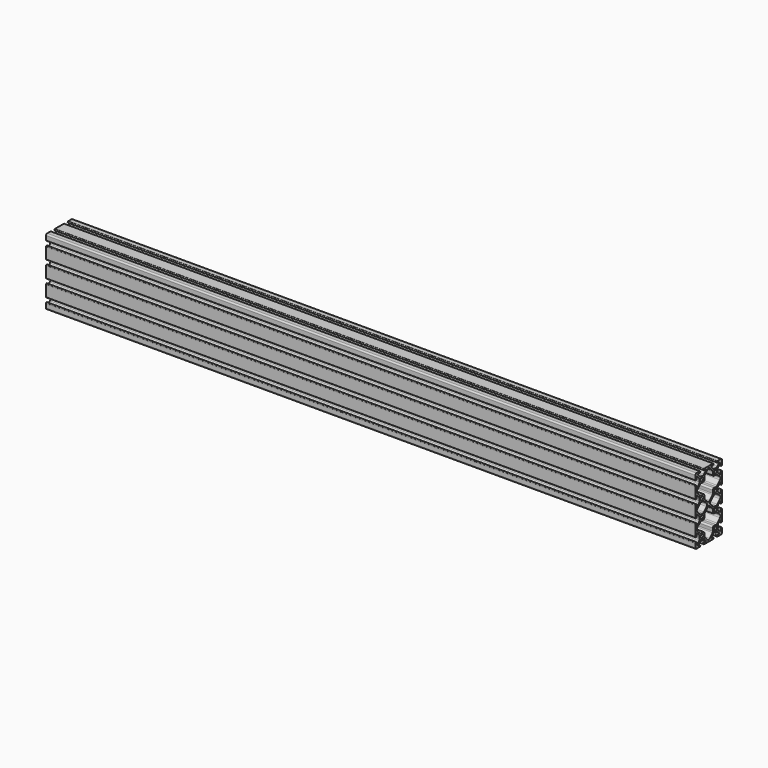
from build123d import *

# Parameters (mm, degrees)
F0_R     = 2.6035
F1_DEPTH = 495.3


# Not quite as in the source:
# - ends of sketch curves that miss each other by under 0.0002 mm in the source are joined


with BuildPart() as f1:
    # F0 (on Right) → F1 (new body, symmetric)
    with BuildSketch(Plane.YZ):
        with BuildLine():
            Line((-130.535426, 44.2699648), (-130.535426, 46.4424522))
            ThreePointArc((-130.535426, 46.4424522), (-131.640326, 47.5473522), (-132.745226, 46.4424522))
            Line((-132.745226, 46.4424522), (-132.745226, 29.6470578))
            ThreePointArc((-132.745226, 29.6470578), (-131.640326, 28.5421578), (-130.535426, 29.6470578))
            Line((-130.535426, 29.6470578), (-130.535426, 31.8195452))
            ThreePointArc((-130.535426, 31.8195452), (-129.9082323673, 32.758206805), (-128.8010055103, 32.5379656897))
            Line((-128.8010055103, 32.5379656897), (-125.4836708, 29.2206172))
            ThreePointArc((-125.4836708, 29.2206172), (-124.7954084843, 28.1905818978), (-124.553726, 26.975562))
            Line((-124.553726, 26.975562), (-124.553726, 23.713948))
            ThreePointArc((-124.553726, 23.713948), (-124.7954084843, 22.4989281022), (-125.4836619697, 21.4688839697))
            Line((-125.4836619697, 21.4688839697), (-128.8010124, 18.1515512))
            ThreePointArc((-128.8010124, 18.1515512), (-129.9082323673, 17.931303195), (-130.535426, 18.8699648))
            Line((-130.535426, 18.8699648), (-130.535426, 21.0424522))
            ThreePointArc((-130.535426, 21.0424522), (-131.640326, 22.1473522), (-132.745226, 21.0424522))
            Line((-132.745226, 21.0424522), (-132.745226, 4.2470578))
            ThreePointArc((-132.745226, 4.2470578), (-131.640326, 3.1421578), (-130.535426, 4.2470578))
            Line((-130.535426, 4.2470578), (-130.535426, 6.4195452))
            ThreePointArc((-130.535426, 6.4195452), (-129.9082323673, 7.358206805), (-128.8010055103, 7.1379656897))
            Line((-128.8010055103, 7.1379656897), (-125.4836708, 3.8206172))
            ThreePointArc((-125.4836708, 3.8206172), (-124.7954084843, 2.7905818978), (-124.553726, 1.575562))
            Line((-124.553726, 1.575562), (-124.553726, -1.686052))
            ThreePointArc((-124.553726, -1.686052), (-124.7954084843, -2.9010718978), (-125.4836619697, -3.9311160303))
            Line((-125.4836619697, -3.9311160303), (-128.8010124, -7.2484488))
            ThreePointArc((-128.8010124, -7.2484488), (-129.9082323673, -7.468696805), (-130.535426, -6.5300352))
            Line((-130.535426, -6.5300352), (-130.535426, -4.3575478))
            ThreePointArc((-130.535426, -4.3575478), (-131.640326, -3.2526478), (-132.745226, -4.3575478))
            Line((-132.745226, -4.3575478), (-132.7452382396, -10.634344926))
            ThreePointArc((-132.7452382396, -10.634344926), (-132.1277993161, -12.1378183161), (-130.624325926, -12.7552572396))
            Line((-130.624325926, -12.7552572396), (-124.3475288, -12.755245))
            ThreePointArc((-124.3475288, -12.755245), (-123.2426288, -11.650345), (-124.3475288, -10.545445))
            Line((-124.3475288, -10.545445), (-126.5200162, -10.545445))
            ThreePointArc((-126.5200162, -10.545445), (-127.458677805, -9.9182513673), (-127.2384366897, -8.8110245103))
            Line((-127.2384366897, -8.8110245103), (-123.9210882, -5.4936898))
            ThreePointArc((-123.9210882, -5.4936898), (-122.8910528978, -4.8054274843), (-121.676033, -4.563745))
            Line((-121.676033, -4.563745), (-118.414419, -4.563745))
            ThreePointArc((-118.414419, -4.563745), (-117.1993991022, -4.8054274843), (-116.1693549697, -5.4936809697))
            Line((-116.1693549697, -5.4936809697), (-112.8520222, -8.8110314))
            ThreePointArc((-112.8520222, -8.8110314), (-112.631774195, -9.9182513673), (-113.5704358, -10.545445))
            Line((-113.5704358, -10.545445), (-115.7429232, -10.545445))
            ThreePointArc((-115.7429232, -10.545445), (-116.8478232, -11.650345), (-115.7429232, -12.755245))
            Line((-115.7429232, -12.755245), (-98.9475288, -12.755245))
            ThreePointArc((-98.9475288, -12.755245), (-97.8426288, -11.650345), (-98.9475288, -10.545445))
            Line((-98.9475288, -10.545445), (-101.1200162, -10.545445))
            ThreePointArc((-101.1200162, -10.545445), (-102.058677805, -9.9182513673), (-101.8384366897, -8.8110245103))
            Line((-101.8384366897, -8.8110245103), (-98.5210882, -5.4936898))
            ThreePointArc((-98.5210882, -5.4936898), (-97.4910528978, -4.8054274843), (-96.276033, -4.563745))
            Line((-96.276033, -4.563745), (-93.014419, -4.563745))
            ThreePointArc((-93.014419, -4.563745), (-91.7993991022, -4.8054274843), (-90.7693549697, -5.4936809697))
            Line((-90.7693549697, -5.4936809697), (-87.4520222, -8.8110314))
            ThreePointArc((-87.4520222, -8.8110314), (-87.231774195, -9.9182513673), (-88.1704358, -10.545445))
            Line((-88.1704358, -10.545445), (-90.3429232, -10.545445))
            ThreePointArc((-90.3429232, -10.545445), (-91.4478232, -11.650345), (-90.3429232, -12.755245))
            Line((-90.3429232, -12.755245), (-84.066126074, -12.7552572396))
            ThreePointArc((-84.066126074, -12.7552572396), (-82.5626526839, -12.1378183161), (-81.9452137604, -10.634344926))
            Line((-81.9452137604, -10.634344926), (-81.945226, -4.3575478))
            ThreePointArc((-81.945226, -4.3575478), (-83.050126, -3.2526478), (-84.155026, -4.3575478))
            Line((-84.155026, -4.3575478), (-84.155026, -6.5300352))
            ThreePointArc((-84.155026, -6.5300352), (-84.7822196327, -7.468696805), (-85.8894464897, -7.2484556897))
            Line((-85.8894464897, -7.2484556897), (-89.2067812, -3.9311072))
            ThreePointArc((-89.2067812, -3.9311072), (-89.8950435157, -2.9010718978), (-90.136726, -1.686052))
            Line((-90.136726, -1.686052), (-90.136726, 1.575562))
            ThreePointArc((-90.136726, 1.575562), (-89.8950435157, 2.7905818978), (-89.2067900303, 3.8206260303))
            Line((-89.2067900303, 3.8206260303), (-85.8894396, 7.1379588))
            ThreePointArc((-85.8894396, 7.1379588), (-84.7822196327, 7.358206805), (-84.155026, 6.4195452))
            Line((-84.155026, 6.4195452), (-84.155026, 4.2470578))
            ThreePointArc((-84.155026, 4.2470578), (-83.050126, 3.1421578), (-81.945226, 4.2470578))
            Line((-81.945226, 4.2470578), (-81.945226, 21.0424522))
            ThreePointArc((-81.945226, 21.0424522), (-83.050126, 22.1473522), (-84.155026, 21.0424522))
            Line((-84.155026, 21.0424522), (-84.155026, 18.8699648))
            ThreePointArc((-84.155026, 18.8699648), (-84.7822196327, 17.931303195), (-85.8894464897, 18.1515443103))
            Line((-85.8894464897, 18.1515443103), (-89.2067812, 21.4688928))
            ThreePointArc((-89.2067812, 21.4688928), (-89.8950435157, 22.4989281022), (-90.136726, 23.713948))
            Line((-90.136726, 23.713948), (-90.136726, 26.975562))
            ThreePointArc((-90.136726, 26.975562), (-89.8950435157, 28.1905818978), (-89.2067900303, 29.2206260303))
            Line((-89.2067900303, 29.2206260303), (-85.8894396, 32.5379588))
            ThreePointArc((-85.8894396, 32.5379588), (-84.7822196327, 32.758206805), (-84.155026, 31.8195452))
            Line((-84.155026, 31.8195452), (-84.155026, 29.6470578))
            ThreePointArc((-84.155026, 29.6470578), (-83.050126, 28.5421578), (-81.945226, 29.6470578))
            Line((-81.945226, 29.6470578), (-81.945226, 46.4424522))
            ThreePointArc((-81.945226, 46.4424522), (-83.050126, 47.5473522), (-84.155026, 46.4424522))
            Line((-84.155026, 46.4424522), (-84.155026, 44.2699648))
            ThreePointArc((-84.155026, 44.2699648), (-84.7822196327, 43.331303195), (-85.8894464897, 43.5515443103))
            Line((-85.8894464897, 43.5515443103), (-89.2067812, 46.8688928))
            ThreePointArc((-89.2067812, 46.8688928), (-89.8950435157, 47.8989281022), (-90.136726, 49.113948))
            Line((-90.136726, 49.113948), (-90.1367316114, 52.375562))
            ThreePointArc((-90.1367316114, 52.375562), (-89.8950435157, 53.5905818978), (-89.2067900303, 54.6206260303))
            Line((-89.2067900303, 54.6206260303), (-85.8894396, 57.9379588))
            ThreePointArc((-85.8894396, 57.9379588), (-84.7822196327, 58.158206805), (-84.155026, 57.2195452))
            Line((-84.155026, 57.2195452), (-84.155026, 55.0470578))
            ThreePointArc((-84.155026, 55.0470578), (-83.0501583484, 53.9421578), (-81.9452583484, 55.0470578))
            Line((-81.9452583484, 55.0470578), (-81.9452255979, 71.8424522))
            ThreePointArc((-81.9452255979, 71.8424522), (-83.0501255979, 72.9473522), (-84.1550255979, 71.8424522))
            Line((-84.1550255979, 71.8424522), (-84.155026, 69.6699648))
            ThreePointArc((-84.155026, 69.6699648), (-84.7822196327, 68.731303195), (-85.8894464897, 68.9515443103))
            Line((-85.8894464897, 68.9515443103), (-89.2067812, 72.2688928))
            ThreePointArc((-89.2067812, 72.2688928), (-89.8950435157, 73.2989281022), (-90.136726, 74.513948))
            Line((-90.136726, 74.513948), (-90.1367316114, 77.775562))
            ThreePointArc((-90.1367316114, 77.775562), (-89.8950435157, 78.9905818978), (-89.2067900303, 80.0206260303))
            Line((-89.2067900303, 80.0206260303), (-85.8894396, 83.3379588))
            ThreePointArc((-85.8894396, 83.3379588), (-84.7822196327, 83.558206805), (-84.155026, 82.6195452))
            Line((-84.155026, 82.6195452), (-84.155026, 80.4470578))
            ThreePointArc((-84.155026, 80.4470578), (-83.050126, 79.3421578), (-81.945226, 80.4470578))
            Line((-81.945226, 80.4470578), (-81.9452137604, 86.723854926))
            ThreePointArc((-81.9452137604, 86.723854926), (-82.5626526839, 88.2273283161), (-84.066126074, 88.8447672396))
            Line((-84.066126074, 88.8447672396), (-90.3429232, 88.844755))
            ThreePointArc((-90.3429232, 88.844755), (-91.4478232, 87.739855), (-90.3429232, 86.634955))
            Line((-90.3429232, 86.634955), (-88.1704358, 86.634955))
            ThreePointArc((-88.1704358, 86.634955), (-87.231774195, 86.0077613673), (-87.4520153103, 84.9005345103))
            Line((-87.4520153103, 84.9005345103), (-90.7693638, 81.5831998))
            ThreePointArc((-90.7693638, 81.5831998), (-91.7993991022, 80.8949374843), (-93.014419, 80.653255))
            Line((-93.014419, 80.653255), (-96.276033, 80.6532829446))
            ThreePointArc((-96.276033, 80.6532829446), (-97.4910528978, 80.8949374843), (-98.5210970303, 81.5831909697))
            Line((-98.5210970303, 81.5831909697), (-101.8384298, 84.9005414))
            ThreePointArc((-101.8384298, 84.9005414), (-102.058677805, 86.0077613673), (-101.1200162, 86.634955))
            Line((-101.1200162, 86.634955), (-98.9475288, 86.634955))
            ThreePointArc((-98.9475288, 86.634955), (-97.8426288, 87.739855), (-98.9475288, 88.844755))
            Line((-98.9475288, 88.844755), (-115.7429232, 88.844755))
            ThreePointArc((-115.7429232, 88.844755), (-116.8478232, 87.739855), (-115.7429232, 86.634955))
            Line((-115.7429232, 86.634955), (-113.5704358, 86.634955))
            ThreePointArc((-113.5704358, 86.634955), (-112.631774195, 86.0077613673), (-112.8520153103, 84.9005345103))
            Line((-112.8520153103, 84.9005345103), (-116.1693638, 81.5831998))
            ThreePointArc((-116.1693638, 81.5831998), (-117.1993991022, 80.8949374843), (-118.414419, 80.653255))
            Line((-118.414419, 80.653255), (-121.676033, 80.6532765846))
            ThreePointArc((-121.676033, 80.6532765846), (-122.8910528978, 80.8949374843), (-123.9210970303, 81.5831909697))
            Line((-123.9210970303, 81.5831909697), (-127.2384298, 84.9005414))
            ThreePointArc((-127.2384298, 84.9005414), (-127.458677805, 86.0077613673), (-126.5200162, 86.634955))
            Line((-126.5200162, 86.634955), (-124.3475288, 86.634955))
            ThreePointArc((-124.3475288, 86.634955), (-123.2426288, 87.739855), (-124.3475288, 88.844755))
            Line((-124.3475288, 88.844755), (-130.624325926, 88.8447672396))
            ThreePointArc((-130.624325926, 88.8447672396), (-132.1277993161, 88.2273283161), (-132.7452382396, 86.723854926))
            Line((-132.7452382396, 86.723854926), (-132.745226, 80.4470578))
            ThreePointArc((-132.745226, 80.4470578), (-131.640326, 79.3421578), (-130.535426, 80.4470578))
            Line((-130.535426, 80.4470578), (-130.535426, 82.6195452))
            ThreePointArc((-130.535426, 82.6195452), (-129.9082323673, 83.558206805), (-128.8010055103, 83.3379656897))
            Line((-128.8010055103, 83.3379656897), (-125.4836708, 80.0206172))
            ThreePointArc((-125.4836708, 80.0206172), (-124.7954084843, 78.9905818978), (-124.553726, 77.775562))
            Line((-124.553726, 77.775562), (-124.553726, 74.513948))
            ThreePointArc((-124.553726, 74.513948), (-124.7954084843, 73.2989281022), (-125.4836619697, 72.2688839697))
            Line((-125.4836619697, 72.2688839697), (-128.8010124, 68.9515512))
            ThreePointArc((-128.8010124, 68.9515512), (-129.9082323673, 68.731303195), (-130.535426, 69.6699648))
            Line((-130.535426, 69.6699648), (-130.535426, 71.8424522))
            ThreePointArc((-130.535426, 71.8424522), (-131.640326, 72.9473522), (-132.745226, 71.8424522))
            Line((-132.745226, 71.8424522), (-132.745226, 55.0470578))
            ThreePointArc((-132.745226, 55.0470578), (-131.640326, 53.9421578), (-130.535426, 55.0470578))
            Line((-130.535426, 55.0470578), (-130.535426, 57.2195452))
            ThreePointArc((-130.535426, 57.2195452), (-129.9082323673, 58.158206805), (-128.8010055103, 57.9379656897))
            Line((-128.8010055103, 57.9379656897), (-125.4836708, 54.6206172))
            ThreePointArc((-125.4836708, 54.6206172), (-124.7954084843, 53.5905818978), (-124.553726, 52.375562))
            Line((-124.553726, 52.375562), (-124.553726, 49.113948))
            ThreePointArc((-124.553726, 49.113948), (-124.7954084843, 47.8989281022), (-125.4836619697, 46.8688839697))
            Line((-125.4836619697, 46.8688839697), (-128.8010124, 43.5515512))
            ThreePointArc((-128.8010124, 43.5515512), (-129.9082323673, 43.331303195), (-130.535426, 44.2699648))
        make_face()
        with Locations((-120.045226, -0.055245)):
            Circle(F0_R, mode=Mode.SUBTRACT)
        with BuildLine():
            ThreePointArc((-109.4106849078, 34.4167277078), (-108.4630443059, 35.0499209145), (-107.345226, 35.2722688))
            ThreePointArc((-107.345226, 35.2722688), (-106.2274076941, 35.0499209145), (-105.2797670922, 34.4167277078))
            Line((-105.2797670922, 34.4167277078), (-99.8009688, 28.9379152))
            ThreePointArc((-99.8009688, 28.9379152), (-99.3219370091, 28.2210118488), (-99.153726, 27.375358))
            Line((-99.153726, 27.375358), (-99.153726, 23.046055))
            ThreePointArc((-99.153726, 23.046055), (-98.5064905651, 21.4834904349), (-96.943926, 20.836255))
            Line((-96.943926, 20.836255), (-93.014419, 20.836255))
            ThreePointArc((-93.014419, 20.836255), (-91.7993991022, 20.5945725157), (-90.7693549697, 19.9063190303))
            Line((-90.7693549697, 19.9063190303), (-85.5732604, 14.7102068))
            ThreePointArc((-85.5732604, 14.7102068), (-84.7177122, 12.644755), (-85.5732532922, 10.5792960922))
            Line((-85.5732532922, 10.5792960922), (-90.7693638, 5.3831998))
            ThreePointArc((-90.7693638, 5.3831998), (-91.7993991022, 4.6949374843), (-93.014419, 4.453255))
            Line((-93.014419, 4.453255), (-96.943926, 4.453255))
            ThreePointArc((-96.943926, 4.453255), (-98.5064905651, 3.8060195651), (-99.153726, 2.243455))
            Line((-99.153726, 2.243455), (-99.153726, -2.085848))
            ThreePointArc((-99.153726, -2.085848), (-99.3219370091, -2.9315018488), (-99.8009614349, -3.6484125651))
            Line((-99.8009614349, -3.6484125651), (-105.2797742, -9.1272106))
            ThreePointArc((-105.2797742, -9.1272106), (-107.345226, -9.9827588), (-109.4106849078, -9.1272177078))
            Line((-109.4106849078, -9.1272177078), (-114.8894832, -3.6484052))
            ThreePointArc((-114.8894832, -3.6484052), (-115.3685149909, -2.9315018488), (-115.536726, -2.085848))
            Line((-115.536726, -2.085848), (-115.536726, 2.243455))
            ThreePointArc((-115.536726, 2.243455), (-116.1839614349, 3.8060195651), (-117.746526, 4.453255))
            Line((-117.746526, 4.453255), (-121.676033, 4.453255))
            ThreePointArc((-121.676033, 4.453255), (-122.8910528978, 4.6949374843), (-123.9210970303, 5.3831909697))
            Line((-123.9210970303, 5.3831909697), (-129.1171916, 10.5793032))
            ThreePointArc((-129.1171916, 10.5793032), (-129.9727398, 12.644755), (-129.1171987078, 14.7102139078))
            Line((-129.1171987078, 14.7102139078), (-123.9210882, 19.9063102))
            ThreePointArc((-123.9210882, 19.9063102), (-122.8910528978, 20.5945725157), (-121.676033, 20.836255))
            Line((-121.676033, 20.836255), (-117.746526, 20.836255))
            ThreePointArc((-117.746526, 20.836255), (-116.1839614349, 21.4834904349), (-115.536726, 23.046055))
            Line((-115.536726, 23.046055), (-115.536726, 27.375358))
            ThreePointArc((-115.536726, 27.375358), (-115.3685149909, 28.2210118488), (-114.8894905651, 28.9379225651))
            Line((-114.8894905651, 28.9379225651), (-109.4106849078, 34.4167277078))
        make_face(mode=Mode.SUBTRACT)
        with Locations((-120.045226, 25.344755)):
            Circle(F0_R, mode=Mode.SUBTRACT)
        with BuildLine():
            ThreePointArc((-123.9210970303, 45.3063190303), (-122.8910528978, 45.9945725157), (-121.676033, 46.236255))
            Line((-121.676033, 46.236255), (-118.414419, 46.236255))
            ThreePointArc((-118.414419, 46.236255), (-117.1993991022, 45.9945725157), (-116.1693549697, 45.3063190303))
            Line((-116.1693549697, 45.3063190303), (-110.9732604, 40.1102068))
            ThreePointArc((-110.9732604, 40.1102068), (-110.1177122, 38.044755), (-110.9732532922, 35.9792960922))
            Line((-110.9732532922, 35.9792960922), (-116.1693638, 30.7831998))
            ThreePointArc((-116.1693638, 30.7831998), (-117.1993991022, 30.0949374843), (-118.414419, 29.853255))
            Line((-118.414419, 29.853255), (-121.676033, 29.853255))
            ThreePointArc((-121.676033, 29.853255), (-122.8910528978, 30.0949374843), (-123.9210970303, 30.7831909697))
            Line((-123.9210970303, 30.7831909697), (-129.1171916, 35.9793032))
            ThreePointArc((-129.1171916, 35.9793032), (-129.9727398, 38.044755), (-129.1171987078, 40.1102139078))
            Line((-129.1171987078, 40.1102139078), (-123.9210970303, 45.3063190303))
        make_face(mode=Mode.SUBTRACT)
        with Locations((-94.645226, -0.055245)):
            Circle(F0_R, mode=Mode.SUBTRACT)
        with Locations((-94.645226, 25.344755)):
            Circle(F0_R, mode=Mode.SUBTRACT)
        with Locations((-120.045226, 50.744755)):
            Circle(F0_R, mode=Mode.SUBTRACT)
        with BuildLine():
            ThreePointArc((-123.9210970303, 70.7063190303), (-122.8910528978, 71.3945725157), (-121.676033, 71.636255))
            Line((-121.676033, 71.636255), (-117.746526, 71.636255))
            ThreePointArc((-117.746526, 71.636255), (-116.1839614349, 72.2834904349), (-115.536726, 73.846055))
            Line((-115.536726, 73.846055), (-115.536726, 78.175358))
            ThreePointArc((-115.536726, 78.175358), (-115.3685149909, 79.0210118488), (-114.8894905651, 79.7379225651))
            Line((-114.8894905651, 79.7379225651), (-109.4106778, 85.2167206))
            ThreePointArc((-109.4106778, 85.2167206), (-107.345226, 86.0722688), (-105.2797670922, 85.2167277078))
            Line((-105.2797670922, 85.2167277078), (-99.8009688, 79.7379152))
            ThreePointArc((-99.8009688, 79.7379152), (-99.3219370091, 79.0210118488), (-99.153726, 78.175358))
            Line((-99.153726, 78.175358), (-99.153721691, 73.846055))
            ThreePointArc((-99.153721691, 73.846055), (-98.5064905651, 72.2834904349), (-96.943926, 71.636255))
            Line((-96.943926, 71.636255), (-93.014419, 71.6362606114))
            ThreePointArc((-93.014419, 71.6362606114), (-91.7993991022, 71.3945725157), (-90.7693549697, 70.7063190303))
            Line((-90.7693549697, 70.7063190303), (-85.5732604, 65.5102068))
            ThreePointArc((-85.5732604, 65.5102068), (-84.7177122, 63.444755), (-85.5732532922, 61.3792960922))
            Line((-85.5732532922, 61.3792960922), (-90.7693638, 56.1831998))
            ThreePointArc((-90.7693638, 56.1831998), (-91.7993991022, 55.4949374843), (-93.014419, 55.253255))
            Line((-93.014419, 55.253255), (-96.943926, 55.2532842469))
            ThreePointArc((-96.943926, 55.2532842469), (-98.5064905651, 54.6060195651), (-99.153726, 53.043455))
            Line((-99.153726, 53.043455), (-99.153726, 48.714152))
            ThreePointArc((-99.153726, 48.714152), (-99.3219370091, 47.8684981512), (-99.8009614349, 47.1515874349))
            Line((-99.8009614349, 47.1515874349), (-105.2797742, 41.6727894))
            ThreePointArc((-105.2797742, 41.6727894), (-106.2274076941, 41.0395890855), (-107.345226, 40.8172412))
            ThreePointArc((-107.345226, 40.8172412), (-108.4630443059, 41.0395890855), (-109.4106849078, 41.6727822922))
            Line((-109.4106849078, 41.6727822922), (-114.8894832, 47.1515948))
            ThreePointArc((-114.8894832, 47.1515948), (-115.3685149909, 47.8684981512), (-115.536726, 48.714152))
            Line((-115.536726, 48.714152), (-115.536726, 53.043455))
            ThreePointArc((-115.536726, 53.043455), (-116.1839614349, 54.6060195651), (-117.746526, 55.253255))
            Line((-117.746526, 55.253255), (-121.676033, 55.253255))
            ThreePointArc((-121.676033, 55.253255), (-122.8910528978, 55.4949374843), (-123.9210970303, 56.1831909697))
            Line((-123.9210970303, 56.1831909697), (-129.1171916, 61.3793032))
            ThreePointArc((-129.1171916, 61.3793032), (-129.9727398, 63.444755), (-129.1171987078, 65.5102139078))
            Line((-129.1171987078, 65.5102139078), (-123.9210970303, 70.7063190303))
        make_face(mode=Mode.SUBTRACT)
        with Locations((-120.045226, 76.144755)):
            Circle(F0_R, mode=Mode.SUBTRACT)
        with BuildLine():
            ThreePointArc((-98.5210970303, 45.3063190303), (-97.4910528978, 45.9945725157), (-96.276033, 46.236255))
            Line((-96.276033, 46.236255), (-93.014419, 46.2362765845))
            ThreePointArc((-93.014419, 46.2362765845), (-91.7993991022, 45.9945725157), (-90.7693549697, 45.3063190303))
            Line((-90.7693549697, 45.3063190303), (-85.5732604, 40.1102068))
            ThreePointArc((-85.5732604, 40.1102068), (-84.7177122, 38.044755), (-85.5732532922, 35.9792960922))
            Line((-85.5732532922, 35.9792960922), (-90.7693638, 30.7831998))
            ThreePointArc((-90.7693638, 30.7831998), (-91.7993991022, 30.0949374843), (-93.014419, 29.853255))
            Line((-93.014419, 29.853255), (-96.276033, 29.853255))
            ThreePointArc((-96.276033, 29.853255), (-97.4910528978, 30.0949374843), (-98.5210970303, 30.7831909697))
            Line((-98.5210970303, 30.7831909697), (-103.7171916, 35.9793032))
            ThreePointArc((-103.7171916, 35.9793032), (-104.5727398, 38.044755), (-103.7171987078, 40.1102139078))
            Line((-103.7171987078, 40.1102139078), (-98.5210970303, 45.3063190303))
        make_face(mode=Mode.SUBTRACT)
        with Locations((-94.645226, 50.744755)):
            Circle(F0_R, mode=Mode.SUBTRACT)
        with Locations((-94.645226, 76.144755)):
            Circle(F0_R, mode=Mode.SUBTRACT)
    extrude(amount=F1_DEPTH, both=True)


solid = f1.part
